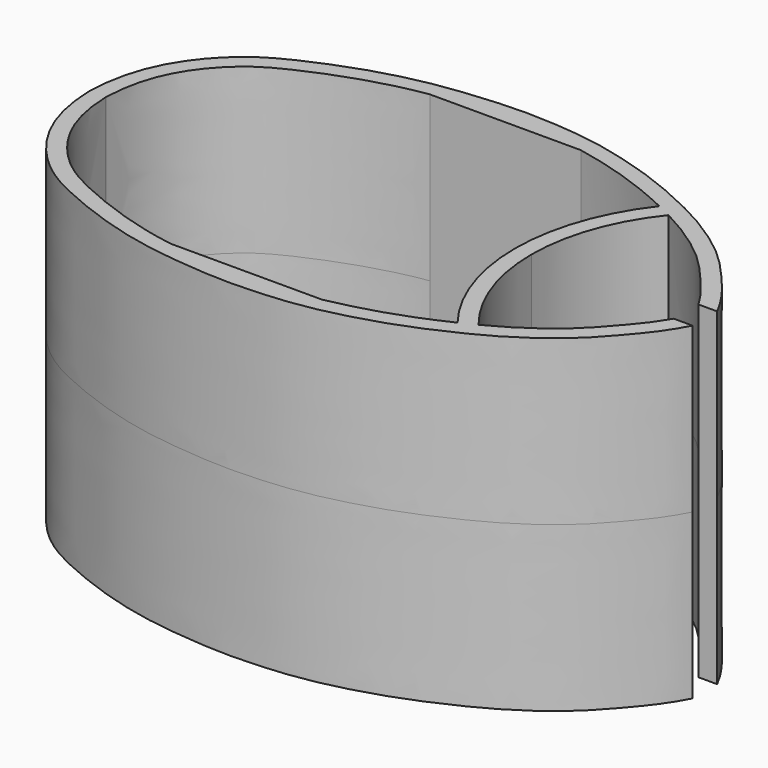
from build123d import *

# Parameters (mm, degrees)
F19_DEPTH = 25.4


# Not quite as in the source:
# - ends of sketch curves that miss each other by under 0.0002 mm in the source are joined
# - the dataset's text gives a spline's control points without its knots; the knots are read off the source's solid


with BuildPart() as f19:
    # F18 (on Top) → F19 (new body, symmetric)
    with BuildSketch(Plane.XY):
        with BuildLine():
            Line((-43.815, 0), (-41.274364031, 0))
            Line((-41.274364031, 0), (-41.274364031, 0.0107594472))
            add(Edge.make_bspline(
                [(-41.274364031, 0.0107594472), (-41.2477378711, 1.3661596464), (-41.0461105432, 3.3581416359), (-40.4801466689, 5.8466573854), (-39.9119087851, 7.6163003428), (-39.2093555266, 9.2678119356), (-38.3748806106, 10.8239592565), (-37.4139591197, 12.2937284374), (-36.3267110013, 13.6931162157), (-35.132922694, 15.0055835598), (-33.8536965602, 16.2044904338), (-32.7323620837, 17.0926256482), (-31.8144631315, 17.7247613585), (-30.8637995003, 18.320756782), (-29.6198390803, 19.0061104284), (-28.309584962, 19.6379349174), (-27.2282396619, 20.1273797903), (-26.1304699992, 20.6115762704), (-24.7648344807, 21.1913224862), (-23.0868238206, 21.8552392863), (-21.3347237158, 22.4913734007), (-19.4620491678, 23.1069136256), (-17.4937213532, 23.686204789), (-15.4662009879, 24.2102580953), (-13.7572955835, 24.586132952), (-12.3927559261, 24.8420192302), (-11.6375273995, 24.9686838433), (-11.2253951687, 25.0334630626), (-11.1550271773, 25.0444)],
                knots=[0.0004181716, 0.0004181716, 0.0004181716, 0.0004181716, 0.03125, 0.046875, 0.0625, 0.078125, 0.09375, 0.109375, 0.125, 0.140625, 0.15625, 0.171875, 0.1796875, 0.1875, 0.203125, 0.21875, 0.2265625, 0.234375, 0.25, 0.265625, 0.28125, 0.296875, 0.3125, 0.328125, 0.34375, 0.3515625, 0.359375, 0.3609843483, 0.3609843483, 0.3609843483, 0.3609843483], degree=3))
            add(Edge.make_bspline(
                [(-11.1550271773, 25.0444), (-10.542199434, 25.1396486856), (-9.2507341781, 25.3205491936), (-7.3235060256, 25.5409372807), (-5.4062672912, 25.7225029254), (-3.6259707874, 25.8679167236), (-1.9439119364, 25.9703614265), (-0.3024423735, 26.0267386411), (1.3666901148, 26.0318853631), (3.0841459509, 25.9889379786), (4.8358815804, 25.9022176908), (6.6182508403, 25.7782185761), (8.3995657193, 25.6136085287), (10.204227939, 25.3891398197), (11.4811176273, 25.1813705052), (12.1601242469, 25.054374244), (12.212939209, 25.0444)],
                knots=[0.3609843483, 0.3609843483, 0.3609843483, 0.3609843483, 0.375, 0.390625, 0.40625, 0.421875, 0.4375, 0.453125, 0.46875, 0.484375, 0.5, 0.515625, 0.53125, 0.546875, 0.5625, 0.5638155672, 0.5638155672, 0.5638155672, 0.5638155672], degree=3))
            add(Edge.make_bspline(
                [(12.212939209, 25.0444), (12.7874079098, 24.935910081), (14.0101485763, 24.6812380165), (15.9013332093, 24.223185306), (17.8100208417, 23.7035416368), (19.6174982681, 23.1637186381), (21.2739675555, 22.6248092168), (22.8673765228, 22.055473021), (24.4716753523, 21.4292847031), (26.1728368077, 20.713506069), (27.630108265, 20.0623448256), (28.4926410945, 19.6608053042), (28.7844012144, 19.5230914963)],
                knots=[0.5638155672, 0.5638155672, 0.5638155672, 0.5638155672, 0.578125, 0.59375, 0.609375, 0.625, 0.640625, 0.65625, 0.671875, 0.6875, 0.703125, 0.7112622913, 0.7112622913, 0.7112622913, 0.7112622913], degree=3))
            add(Edge.make_bspline(
                [(28.7844012144, 19.5230914963), (29.0528707495, 19.3963710863), (29.5952084994, 19.137073037), (30.3776220144, 18.752869828), (30.8778676399, 18.5002539174), (31.1178905157, 18.3771670078)],
                knots=[0.7112622913, 0.7112622913, 0.7112622913, 0.7112622913, 0.71875, 0.7265625, 0.7341002498, 0.7341002498, 0.7341002498, 0.7341002498], degree=3))
            add(Edge.make_bspline(
                [(31.1178905157, 18.3771670078), (31.1266393253, 18.3726805023), (31.632499174, 18.1131209993), (32.5860521639, 17.6068316634), (33.7115864947, 16.9611680115), (34.6154219638, 16.4106109289), (35.5367313786, 15.8276579527), (36.7144333728, 15.0415250136), (37.8645154123, 14.2159344045), (38.733972339, 13.5528506756), (39.5550337441, 12.8979203915), (40.4855128205, 12.0966248777), (41.5131824676, 11.1216924507), (42.5070446229, 10.0950657817), (43.5081058577, 8.991562716), (44.3308167156, 8.0416058596), (44.976892336, 7.278340365), (45.6121545757, 6.5202886328), (46.2066805308, 5.793426823), (46.7687995513, 5.0673381808), (47.1761207946, 4.5162992747), (47.5696893531, 3.9537164713), (47.9591886693, 3.3617532401), (48.2891878893, 2.8316504671), (48.4790184853, 2.5122153516), (48.5516575282, 2.3875989692)],
                knots=[0.7341002498, 0.7341002498, 0.7341002498, 0.7341002498, 0.734375, 0.75, 0.765625, 0.7734375, 0.78125, 0.796875, 0.8125, 0.8203125, 0.828125, 0.84375, 0.859375, 0.875, 0.890625, 0.90625, 0.9140625, 0.921875, 0.9375, 0.9453125, 0.953125, 0.9609375, 0.96875, 0.9765625, 0.9817935421, 0.9817935421, 0.9817935421, 0.9817935421], degree=3))
            Line((48.5516575282, 2.3875989692), (51.435, 2.3875989692))
            add(Edge.make_bspline(
                [(-43.815, 0), (-43.7624752522, 3.0037439428), (-42.7423638876, 8.5233473205), (-39.0064769176, 14.9202682328), (-33.8586937997, 19.8303271293), (-27.9721607189, 22.6424605748), (-21.8677478175, 25.1331163292), (-13.8004564967, 27.3955304745), (-5.8675891054, 28.2786991968), (-0.0489766797, 28.6604633775), (5.9976629011, 28.4342151338), (12.5436865646, 27.7572763922), (19.9604839819, 25.8056227743), (25.5276133686, 23.8341537712), (31.7366717098, 20.9964428844), (36.2360615235, 18.5041540338), (40.964844667, 15.1817120352), (44.1938244908, 12.1020479683), (47.1235637345, 8.7006128803), (49.599038946, 5.6639958266), (51.0575334731, 3.1755801978), (51.435, 2.3875989692)],
                knots=[0, 0, 0, 0, 0.0621231068, 0.1193322831, 0.1753384592, 0.2290296673, 0.2834569581, 0.3451113152, 0.4051603052, 0.456236404, 0.5078123021, 0.5626531156, 0.6210927937, 0.6732906127, 0.7280860429, 0.7768031474, 0.8272977729, 0.8723835911, 0.9169026962, 0.9599145905, 1, 1, 1, 1], degree=3))
        make_face()
        with BuildLine():
            add(Edge.make_bspline(
                [(-11.1550271773, 25.0444), (-10.542199434, 25.1396486856), (-9.2507341781, 25.3205491936), (-7.3235060256, 25.5409372807), (-5.4062672912, 25.7225029254), (-3.6259707874, 25.8679167236), (-1.9439119364, 25.9703614265), (-0.3024423735, 26.0267386411), (1.3666901148, 26.0318853631), (3.0841459509, 25.9889379786), (4.8358815804, 25.9022176908), (6.6182508403, 25.7782185761), (8.3995657193, 25.6136085287), (10.204227939, 25.3891398197), (11.4811176273, 25.1813705052), (12.1601242469, 25.054374244), (12.212939209, 25.0444)],
                knots=[0.3609843483, 0.3609843483, 0.3609843483, 0.3609843483, 0.375, 0.390625, 0.40625, 0.421875, 0.4375, 0.453125, 0.46875, 0.484375, 0.5, 0.515625, 0.53125, 0.546875, 0.5625, 0.5638155672, 0.5638155672, 0.5638155672, 0.5638155672], degree=3))
            Line((-11.1550271773, 25.0444), (12.212939209, 25.0444))
        make_face()
        with BuildLine():
            add(Edge.make_bspline(
                [(28.7844012144, 19.5230914963), (29.0528707495, 19.3963710863), (29.5952084994, 19.137073037), (30.3776220144, 18.752869828), (30.8778676399, 18.5002539174), (31.1178905157, 18.3771670078)],
                knots=[0.7112622913, 0.7112622913, 0.7112622913, 0.7112622913, 0.71875, 0.7265625, 0.7341002498, 0.7341002498, 0.7341002498, 0.7341002498], degree=3))
            ThreePointArc((28.7844012144, 19.5230914963), (23.7973996556, 10.322298401), (22.0726, 0))
            Line((22.0726, 0), (24.6126, 0))
            ThreePointArc((24.6126, 0), (26.2869080345, 9.7472954188), (31.1178905157, 18.3771670078))
        make_face()
    extrude(amount=F19_DEPTH, both=True)

    # F20: F19 across plane


with BuildPart() as f19_1:
    add(f19.part)
    add(f19.part.mirror(Plane.XZ))


solid = f19_1.part
